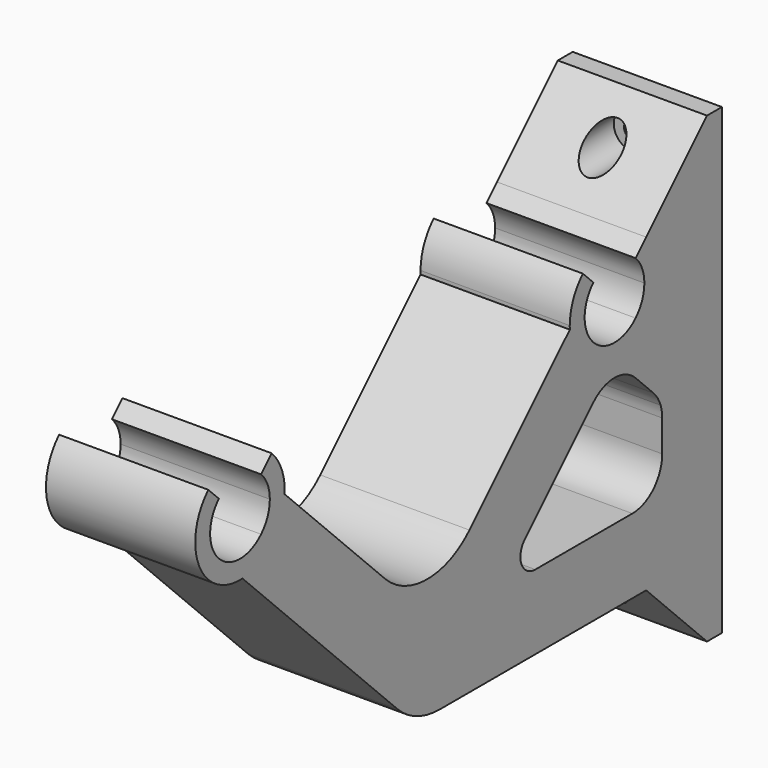
from build123d import *

# Parameters (mm, degrees)
F1_DEPTH = 50.8
F2_R     = 2.8575
F3_DEPTH = 224.1419342397
F5_R     = 6.35
F5_R_2   = 2.8575
F6_DEPTH = 217.7919342397


with BuildPart() as f1:
    # F0 (on Right) → F1 (new body)
    with BuildSketch(Plane.YZ):
        with BuildLine():
            Line((-66.2205500581, -66.2205500581), (-70.7106781187, -70.7106781187))
            ThreePointArc((-70.7106781187, -70.7106781187), (-65.8235712608, -75.2811893269), (-60.6417499855, -79.5146411593))
            ThreePointArc((-60.6417499855, -79.5146411593), (-62.1249501408, -72.3194552405), (-66.2205500581, -66.2205500581))
        make_face()
        with BuildLine():
            Line((-60.6704465476, -80.7509096897), (-70.7106781187, -70.7106781187))
            ThreePointArc((-70.7106781187, -70.7106781187), (-67.9576641768, -74.8308546487), (-66.9909342397, -79.6909342397))
            ThreePointArc((-66.9909342397, -79.6909342397), (-67.9576641768, -84.5510138308), (-70.7106781187, -88.6711903608))
            Line((-70.7106781187, -88.6711903608), (-66.2205500581, -93.1613184213))
            ThreePointArc((-66.2205500581, -93.1613184213), (-62.3007430389, -87.4680641731), (-60.6704465476, -80.7509096897))
        make_face()
        with BuildLine():
            ThreePointArc((-60.6417499855, -79.5146411593), (-65.8235712608, -75.2811893269), (-70.7106781187, -70.7106781187))
            Line((-70.7106781187, -70.7106781187), (-60.6704465476, -80.7509096897))
            ThreePointArc((-60.6704465476, -80.7509096897), (-60.648313746, -80.2211273486), (-60.6409342397, -79.6909342397))
            ThreePointArc((-60.6409342397, -79.6909342397), (-60.6411381773, -79.6027867559), (-60.6417499855, -79.5146411593))
        make_face()
        with BuildLine():
            Line((60.6704465476, -80.7509096897), (70.7106781187, -70.7106781187))
            ThreePointArc((70.7106781187, -70.7106781187), (65.8235712608, -75.2811893269), (60.6417499855, -79.5146411593))
            ThreePointArc((60.6417499855, -79.5146411593), (60.6460643138, -80.133008335), (60.6704465476, -80.7509096897))
        make_face()
        with BuildLine():
            ThreePointArc((60.6417499855, -79.5146411593), (65.8235712608, -75.2811893269), (70.7106781187, -70.7106781187))
            Line((70.7106781187, -70.7106781187), (66.2205500581, -66.2205500581))
            ThreePointArc((66.2205500581, -66.2205500581), (62.1249501408, -72.3194552405), (60.6417499855, -79.5146411593))
        make_face()
        with BuildLine():
            ThreePointArc((70.7106781187, -88.6711903608), (66.9909342397, -79.6909342397), (70.7106781187, -70.7106781187))
            Line((70.7106781187, -70.7106781187), (60.6704465476, -80.7509096897))
            ThreePointArc((60.6704465476, -80.7509096897), (62.3007430389, -87.4680641731), (66.2205500581, -93.1613184213))
            Line((66.2205500581, -93.1613184213), (70.7106781187, -88.6711903608))
        make_face()
        with BuildLine():
            ThreePointArc((98.7409342397, -79.6909342397), (97.2908393341, -72.4008148532), (93.1613184213, -66.2205500581))
            Line((93.1613184213, -66.2205500581), (88.6711903608, -70.7106781187))
            ThreePointArc((88.6711903608, -70.7106781187), (91.4242043026, -74.8308546487), (92.3909342397, -79.6909342397))
            ThreePointArc((92.3909342397, -79.6909342397), (91.4242043026, -84.5510138308), (88.6711903608, -88.6711903608))
            Line((88.6711903608, -88.6711903608), (93.1613184213, -93.1613184213))
            ThreePointArc((93.1613184213, -93.1613184213), (97.2908393341, -86.9810536263), (98.7409342397, -79.6909342397))
        make_face()
        Polygon((119.05, -40.3318684794), (93.1613184213, -66.2205500581), (125.4, -66.2205500581), (125.4, -40.3318684794), align=None)
        with BuildLine():
            Line((125.4, -66.2205500581), (93.1613184213, -66.2205500581))
            ThreePointArc((93.1613184213, -66.2205500581), (97.2908393341, -72.4008148532), (98.7409342397, -79.6909342397))
            ThreePointArc((98.7409342397, -79.6909342397), (97.2908393341, -86.9810536263), (93.1613184213, -93.1613184213))
            ThreePointArc((93.1613184213, -93.1613184213), (79.6909342397, -98.7409342397), (66.2205500581, -93.1613184213))
            Line((66.2205500581, -93.1613184213), (0, -159.3818684794))
            Line((0, -159.3818684794), (-66.2205500581, -93.1613184213))
            ThreePointArc((-66.2205500581, -93.1613184213), (-71.9138043064, -97.0811254405), (-78.6309587898, -98.7114219318))
            Line((-78.6309587898, -98.7114219318), (-12.7, -164.6423807216))
            ThreePointArc((-12.7, -164.6423807216), (-4.4596469399, -170.1484086052), (5.2605122421, -172.0818684794))
            Line((5.2605122421, -172.0818684794), (93.1613184213, -172.0818684794))
            Line((93.1613184213, -172.0818684794), (125.4, -172.0818684794))
            Line((125.4, -172.0818684794), (125.4, -119.1512092688))
            Line((125.4, -119.1512092688), (125.4, -66.2205500581))
        make_face()
        with BuildLine():
            ThreePointArc((96.2802561211, -114.2407683632), (98.0883415579, -116.5201524195), (99.3302370763, -119.1512092688))
            ThreePointArc((99.3302370763, -119.1512092688), (99.8314406767, -121.1587455105), (100, -123.2210244843))
            Line((100, -123.2210244843), (100, -133.9818684794))
            ThreePointArc((100, -133.9818684794), (96.2802561211, -142.9621246005), (87.3, -146.6818684794))
            Line((87.3, -146.6818684794), (45.9907683632, -146.6818684794))
            ThreePointArc((45.9907683632, -146.6818684794), (40.1241333318, -142.761908275), (41.5006403027, -135.8417404189))
            Line((41.5006403027, -135.8417404189), (70.7106781187, -106.6317026029))
            ThreePointArc((70.7106781187, -106.6317026029), (79.6909342397, -102.911958724), (88.6711903608, -106.6317026029))
            Line((88.6711903608, -106.6317026029), (96.2802561211, -114.2407683632))
        make_face(mode=Mode.SUBTRACT)
        with BuildLine():
            Line((-17.9605122421, -123.4608439952), (-60.6704465476, -80.7509096897))
            ThreePointArc((-60.6704465476, -80.7509096897), (-62.3007430389, -87.4680641731), (-66.2205500581, -93.1613184213))
            Line((-66.2205500581, -93.1613184213), (0, -159.3818684794))
            Line((0, -159.3818684794), (66.2205500581, -93.1613184213))
            ThreePointArc((66.2205500581, -93.1613184213), (62.3007430389, -87.4680641731), (60.6704465476, -80.7509096897))
            Line((60.6704465476, -80.7509096897), (17.9605122421, -123.4608439952))
            ThreePointArc((17.9605122421, -123.4608439952), (0, -130.900331753), (-17.9605122421, -123.4608439952))
        make_face()
        with BuildLine():
            Line((-88.6711903608, -70.7106781187), (-93.1613184213, -66.2205500581))
            ThreePointArc((-93.1613184213, -66.2205500581), (-97.0811254405, -87.4680641731), (-78.6309587898, -98.7114219318))
            Line((-78.6309587898, -98.7114219318), (-88.6711903608, -88.6711903608))
            ThreePointArc((-88.6711903608, -88.6711903608), (-92.3909342397, -79.6909342397), (-88.6711903608, -70.7106781187))
        make_face()
        with BuildLine():
            ThreePointArc((88.6711903608, -88.6711903608), (79.6909342397, -92.3909342397), (70.7106781187, -88.6711903608))
            Line((70.7106781187, -88.6711903608), (66.2205500581, -93.1613184213))
            ThreePointArc((66.2205500581, -93.1613184213), (79.6909342397, -98.7409342397), (93.1613184213, -93.1613184213))
            Line((93.1613184213, -93.1613184213), (88.6711903608, -88.6711903608))
        make_face()
        with BuildLine():
            Line((-66.2205500581, -93.1613184213), (-70.7106781187, -88.6711903608))
            ThreePointArc((-70.7106781187, -88.6711903608), (-79.6909342397, -92.3909342397), (-88.6711903608, -88.6711903608))
            Line((-88.6711903608, -88.6711903608), (-78.6309587898, -98.7114219318))
            ThreePointArc((-78.6309587898, -98.7114219318), (-71.9138043064, -97.0811254405), (-66.2205500581, -93.1613184213))
        make_face()
        Polygon((125.4, -197.9705500581), (125.4, -172.0818684794), (93.1613184213, -172.0818684794), (119.05, -197.9705500581), align=None)
    extrude(amount=F1_DEPTH)

    # F2 (on face) → F3 (cut, through all)
    with BuildSketch(Plane(origin=(0, 125.4, 0), x_dir=(-1, 0, 0), z_dir=(0, 1, 0))):
        with Locations((-25.4, -185.2705500581)):
            Circle(F2_R)
        with Locations((-25.4, -53.0318684794)):
            Circle(F2_R)
    extrude(amount=-F3_DEPTH, mode=Mode.SUBTRACT)

    # F5 (on offset) → F6 (cut, through all)
    with BuildSketch(Plane(origin=(0, 119.05, 0), x_dir=(-1, 0, 0), z_dir=(0, 1, 0))):
        with Locations((-25.4, -53.0318684794)):
            Circle(F5_R)
        with Locations((-25.4, -53.0318684794)):
            Circle(F5_R_2, mode=Mode.SUBTRACT)
        with Locations((-25.4, -185.2705500581)):
            Circle(F5_R)
        with Locations((-25.4, -185.2705500581)):
            Circle(F5_R_2, mode=Mode.SUBTRACT)
    extrude(amount=-F6_DEPTH, mode=Mode.SUBTRACT)


solid = f1.part
